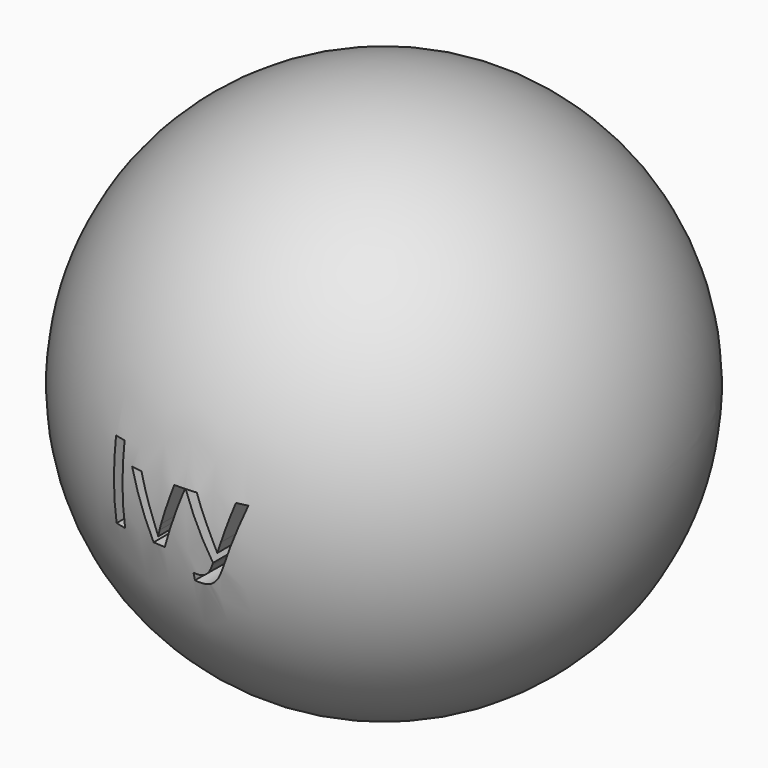
from build123d import *

# Parameters (mm, degrees)
F4_DEPTH = 10
F3_W     = 0.9957388944
F3_H     = 7.3437828345
F5_DEPTH = 10
F6_DEPTH = 10


with BuildPart() as f1:
    # F0 (on Top) → F1 (revolve)
    with BuildSketch(Plane.XY):
        with BuildLine():
            Line((-25, 0), (25, 0))
            ThreePointArc((25, 0), (0, 25), (-25, 0))
        make_face()
    revolve(axis=Axis((0, 0, 0), (-1, 0, 0)))

    # F3 (on offset) → F4 (cut)
    with BuildSketch(Plane.XZ.offset(25)):
        with BuildLine():
            Line((-2.1299138496, -3.89204987), (-1.0190895553, -3.89204987))
            Line((-1.0190895553, -3.89204987), (1.0858057291, 1.7471347231))
            Line((1.0858057291, 1.7471347231), (0.0900668347, 1.7471347231))
            Line((0.0900668347, 1.7471347231), (-1.1908837029, -1.9322622637))
            Line((-1.1908837029, -1.9322622637), (-1.3943680331, -2.5477189673))
            Line((-1.3943680331, -2.5477189673), (-1.5778375111, -3.1565040535))
            add(Edge.make_bspline(
                [(-1.9364369455, -1.9222548377), (-1.8697207716, -2.1307428809), (-1.5778375111, -3.1565040535)],
                knots=[0, 0, 0, 1, 1, 1], degree=2))
            Line((-1.9364369455, -1.9222548377), (-3.1773577787, 1.7471347231))
            Line((-3.1773577787, 1.7471347231), (-4.1781003862, 1.7471347231))
            Line((-4.1781003862, 1.7471347231), (-2.1299138496, -3.89204987))
        make_face()
    extrude(amount=-F4_DEPTH, mode=Mode.SUBTRACT)

    # F3 (on offset) → F5 (cut)
    with BuildSketch(Plane.XZ.offset(25)):
        with Locations((-5.6967272931, -0.2201584528)):
            Rectangle(F3_W, F3_H)
    extrude(amount=-F5_DEPTH, mode=Mode.SUBTRACT)

    # F3 (on offset) → F6 (cut)
    with BuildSketch(Plane.XZ.offset(25)):
        with BuildLine():
            add(Edge.make_bspline(
                [(2.1182385192, -6.1070268413), (1.7329526153, -6.1070268413), (1.471091633, -6.0503180935)],
                knots=[0, 0, 0, 1, 1, 1], degree=2))
            add(Edge.make_bspline(
                [(2.9496888355, -5.8910332285), (2.5819159273, -6.1070268413), (2.1182385192, -6.1070268413)],
                knots=[0, 0, 0, 1, 1, 1], degree=2))
            add(Edge.make_bspline(
                [(3.6193524304, -5.2347128684), (3.3174617438, -5.6750396157), (2.9496888355, -5.8910332285)],
                knots=[0, 0, 0, 1, 1, 1], degree=2))
            add(Edge.make_bspline(
                [(4.2715030296, -3.89204987), (3.921243117, -4.7943861211), (3.6193524304, -5.2347128684)],
                knots=[0, 0, 0, 1, 1, 1], degree=2))
            Line((4.2715030296, -3.89204987), (6.4397786791, 1.7471347231))
            Line((6.4397786791, 1.7471347231), (5.4490434977, 1.7471347231))
            Line((5.4490434977, 1.7471347231), (4.2131263775, -1.8438633334))
            Line((4.2131263775, -1.8438633334), (3.8478553258, -2.8696245061))
            add(Edge.make_bspline(
                [(3.6351975217, -2.2241455242), (3.8328441866, -2.8029083322), (3.8478553258, -2.8696245061)],
                knots=[0, 0, 0, 1, 1, 1], degree=2))
            add(Edge.make_bspline(
                [(3.4008569611, -1.5436405512), (3.4375508567, -1.6453827163), (3.6351975217, -2.2241455242)],
                knots=[0, 0, 0, 1, 1, 1], degree=2))
            add(Edge.make_bspline(
                [(3.3374765959, -1.3685105949), (3.3641630655, -1.4418983861), (3.4008569611, -1.5436405512)],
                knots=[0, 0, 0, 1, 1, 1], degree=2))
            Line((3.3374765959, -1.3685105949), (2.1499287017, 1.7471347231))
            Line((2.1499287017, 1.7471347231), (1.1491860943, 1.7471347231))
            Line((1.1491860943, 1.7471347231), (3.3841779176, -3.8653634005))
            Line((3.3841779176, -3.8653634005), (3.2957789873, -4.0905304872))
            add(Edge.make_bspline(
                [(1.9097504759, -5.3781526422), (2.7854002575, -5.3781526422), (3.2957789873, -4.0905304872)],
                knots=[0, 0, 0, 1, 1, 1], degree=2))
            add(Edge.make_bspline(
                [(1.471091633, -5.3464624596), (1.6695722501, -5.3781526422), (1.9097504759, -5.3781526422)],
                knots=[0, 0, 0, 1, 1, 1], degree=2))
            Line((1.471091633, -5.3464624596), (1.471091633, -6.0503180935))
        make_face()
    extrude(amount=-F6_DEPTH, mode=Mode.SUBTRACT)


solid = f1.part
